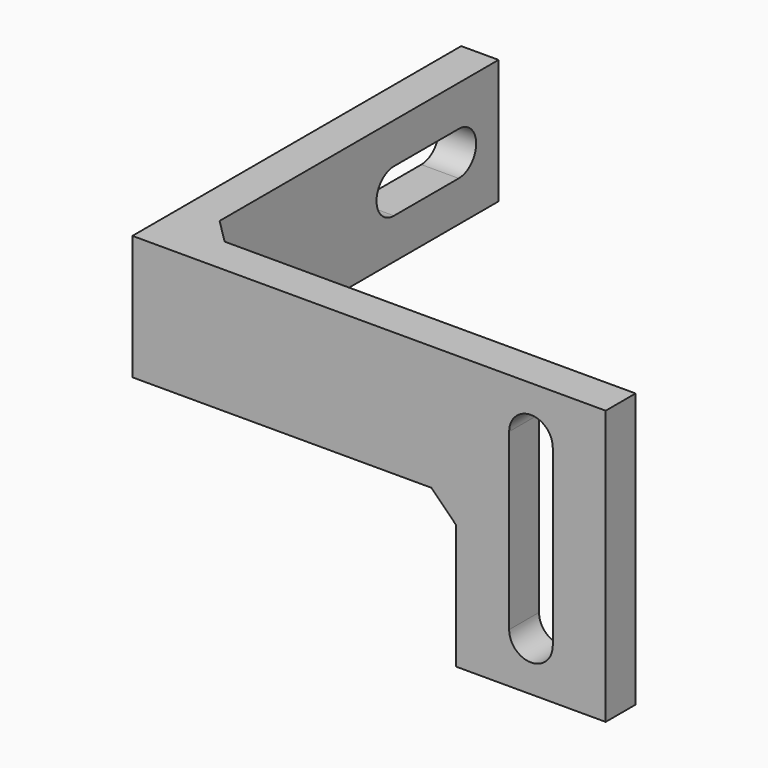
from build123d import *

# Parameters (mm, degrees)
F4_W     = 3
F4_H     = 30
F4_W_2   = 12
F4_H_2   = 3
F5_DEPTH = 10
F0_DEPTH = 12
F2_DEPTH = 38.001
F7_DEPTH = 33.001
F3_SIZE  = 2


# Not quite as in the source:
# - a feature names something its author has since deleted; it is built from what else it names


with BuildPart() as f5:
    # F4 (on Top) → F5 (new body)
    with BuildSketch(Plane.XY):
        with Locations((0, -15)):
            Rectangle(F4_W, F4_H)
        Polygon((1.5, -30), (-1.5, -30), (-1.5, -33), (24.5, -33), (24.5, -30), align=None)
        with Locations((30.5, -31.5)):
            Rectangle(F4_W_2, F4_H_2)
    extrude(amount=F5_DEPTH)

    # F4 (on Top) → F0 (join)
    with BuildSketch(Plane.XY):
        with Locations((30.5, -31.5)):
            Rectangle(F4_W_2, F4_H_2)
    extrude(amount=-F0_DEPTH)

    # F1 (on face) → F2 (cut, through all)
    with BuildSketch(Plane(origin=(-1.5, 0, 0), x_dir=(0, -1, 0), z_dir=(-1, 0, 0))):
        with BuildLine():
            ThreePointArc((4, 3.25), (5.2374368671, 3.7625631329), (5.75, 5))
            ThreePointArc((5.75, 5), (5.2374368671, 6.2374368671), (4, 6.75))
            ThreePointArc((4, 6.75), (2.25, 5), (4, 3.25))
        make_face()
        with BuildLine():
            ThreePointArc((4, 6.75), (5.2374368671, 6.2374368671), (5.75, 5))
            ThreePointArc((5.75, 5), (5.2374368671, 3.7625631329), (4, 3.25))
            Line((4, 3.25), (10.5, 3.25))
            ThreePointArc((10.5, 3.25), (8.75, 5), (10.5, 6.75))
            Line((10.5, 6.75), (4, 6.75))
        make_face()
        with BuildLine():
            ThreePointArc((12.25, 5), (11.7374368671, 6.2374368671), (10.5, 6.75))
            ThreePointArc((10.5, 6.75), (8.75, 5), (10.5, 3.25))
            ThreePointArc((10.5, 3.25), (11.7374368671, 3.7625631329), (12.25, 5))
        make_face()
    extrude(amount=-F2_DEPTH, mode=Mode.SUBTRACT)

    # F6 (on face) → F7 (cut, through all)
    with BuildSketch(Plane.XZ.offset(33)):
        with BuildLine():
            ThreePointArc((28.75, -8), (30.5, -6.25), (32.25, -8))
            Line((32.25, -8), (32.25, 6))
            ThreePointArc((32.25, 6), (30.5, 4.25), (28.75, 6))
            Line((28.75, 6), (28.75, -8))
        make_face()
        with BuildLine():
            ThreePointArc((28.75, -8), (30.5, -9.75), (32.25, -8))
            ThreePointArc((32.25, -8), (30.5, -6.25), (28.75, -8))
        make_face()
        with BuildLine():
            ThreePointArc((28.75, 6), (30.5, 4.25), (32.25, 6))
            ThreePointArc((32.25, 6), (30.5, 7.75), (28.75, 6))
        make_face()
    extrude(amount=-F7_DEPTH, mode=Mode.SUBTRACT)

    # F3
    f3_edges = [f5.edges().sort_by_distance(p)[0] for p in [
        (1.5, -30, 5),
        (24.5, -31.5, 0),
    ]]
    chamfer(f3_edges, length=F3_SIZE)


solid = f5.part
